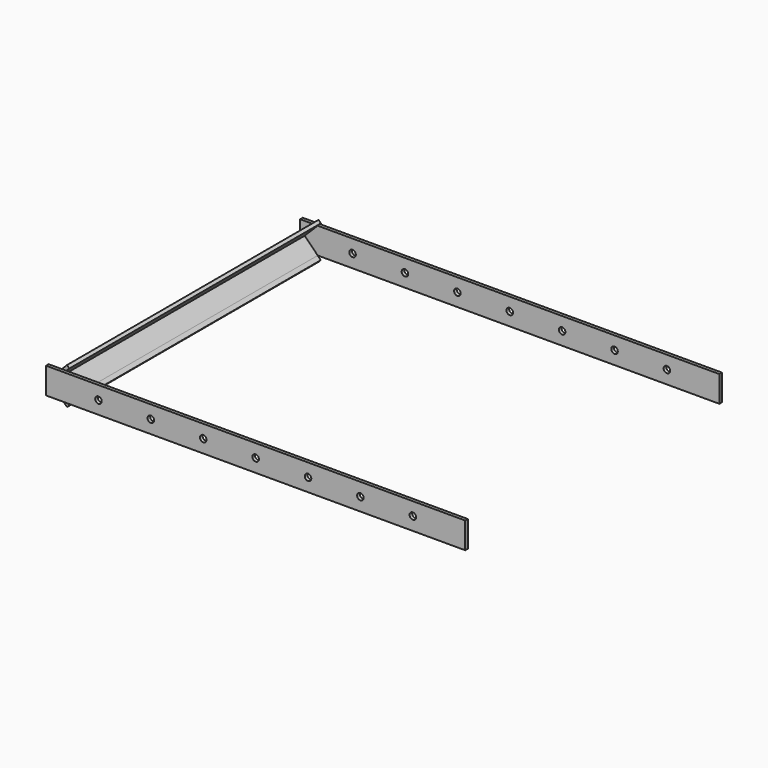
from build123d import *

# Parameters (mm, degrees)
F0_W     = 406.4
F0_H     = 25.4
F0_R     = 3.175
F1_DEPTH = 3.175
F3_DEPTH = 304.8
F4_R     = 3.175
F5_DEPTH = 3.175


# Not quite as in the source:
# - a length typed as a fraction of an inch, garbled in the dataset ("3 / 203.2 mm" for 3/8 in), is restored


with BuildPart() as f1:
    # F0 (on Front) → F1 (new body)
    with BuildSketch(Plane.XZ):
        with Locations((76.9218784556, -2.4463492446)):
            Rectangle(F0_W, F0_H)
        with Locations((-75.4781215444, -2.4463492446)):
            Circle(F0_R, mode=Mode.SUBTRACT)
        with Locations((-24.6781215444, -2.4463492446)):
            Circle(F0_R, mode=Mode.SUBTRACT)
        with Locations((26.1218784556, -2.4463492446)):
            Circle(F0_R, mode=Mode.SUBTRACT)
        with Locations((76.9218784556, -2.4463492446)):
            Circle(F0_R, mode=Mode.SUBTRACT)
        with Locations((127.7218784556, -2.4463492446)):
            Circle(F0_R, mode=Mode.SUBTRACT)
        with Locations((178.5218784556, -2.4463492446)):
            Circle(F0_R, mode=Mode.SUBTRACT)
        with Locations((229.3218784556, -2.4463492446)):
            Circle(F0_R, mode=Mode.SUBTRACT)
    extrude(amount=F1_DEPTH)

    # F2 (on face) → F3 (join)
    with BuildSketch(Plane.XZ.offset(3.175)):
        Polygon((-108.4897565831, 15.5141629976), (-113.7502688252, 10.2536507554), (-109.2601407647, 10.2536507554), (-106.2446925528, 13.2690989673), align=None)
        Polygon((-113.7502688252, 10.2536507554), (-126.2781215444, -2.2742019637), (-126.2781215444, -2.4463492446), (-126.2781215444, -2.6184965255), (-113.7502688252, -15.1463492446), (-109.2601407647, -15.1463492446), (-121.9601407647, -2.4463492446), (-109.2601407647, 10.2536507554), align=None)
        Polygon((-109.2601407647, -15.1463492446), (-113.7502688252, -15.1463492446), (-108.4897565831, -20.4068614867), (-106.2446925528, -18.1617974564), align=None)
    extrude(amount=F3_DEPTH)

    # F4 (on face) → F5 (join)
    with BuildSketch(Plane.XZ.offset(307.975)):
        Polygon((280.1218784556, 10.4257980363), (-109.0879934838, 10.4257980363), (-121.9601407647, -2.4463492446), (-109.4322880456, -14.9742019637), (280.1218784556, -14.9742019637), align=None)
        with Locations((-75.4781215444, -2.4463492446)):
            Circle(F4_R, mode=Mode.SUBTRACT)
        with Locations((-24.6781215444, -2.2742019637)):
            Circle(F4_R, mode=Mode.SUBTRACT)
        with Locations((26.1218784556, -2.2742019637)):
            Circle(F4_R, mode=Mode.SUBTRACT)
        with Locations((76.9218784556, -2.2742019637)):
            Circle(F4_R, mode=Mode.SUBTRACT)
        with Locations((127.7218784556, -2.2742019637)):
            Circle(F4_R, mode=Mode.SUBTRACT)
        with Locations((178.5218784556, -2.2742019637)):
            Circle(F4_R, mode=Mode.SUBTRACT)
        with Locations((229.3218784556, -2.2742019637)):
            Circle(F4_R, mode=Mode.SUBTRACT)
        Polygon((-126.2781215444, 10.4257980363), (-126.2781215444, -2.2742019637), (-113.5781215444, 10.4257980363), align=None)
        Polygon((-113.9224161061, -14.9742019637), (-126.2781215444, -2.6184965255), (-126.2781215444, -14.9742019637), align=None)
        Polygon((-113.5781215444, 10.4257980363), (-126.2781215444, -2.2742019637), (-126.2781215444, -2.6184965255), (-113.9224161061, -14.9742019637), (-109.4322880456, -14.9742019637), (-121.9601407647, -2.4463492446), (-109.0879934838, 10.4257980363), align=None)
    extrude(amount=F5_DEPTH)


solid = f1.part
